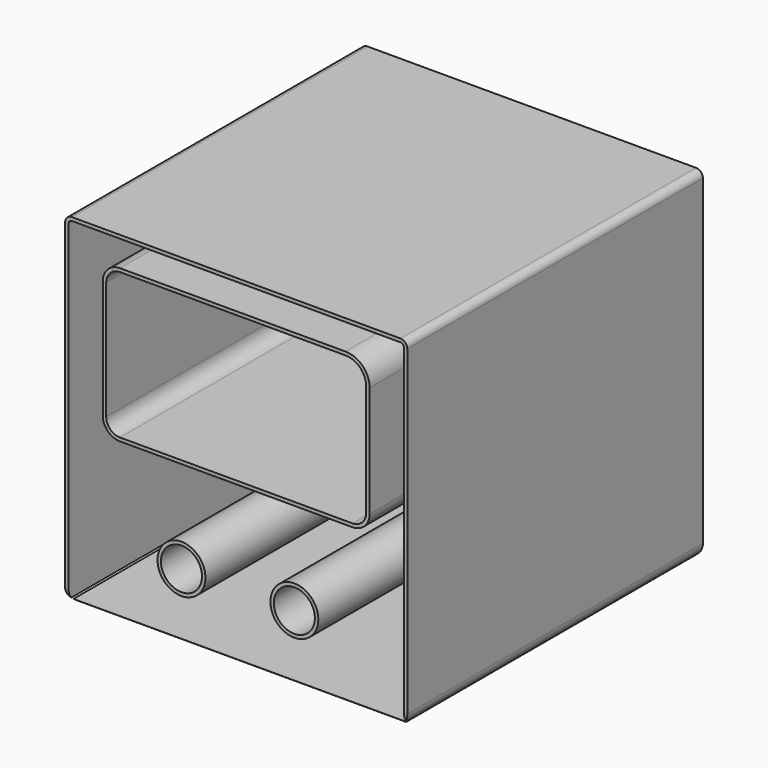
from build123d import *

# Parameters (mm, degrees)
F0_W        = 250
F0_H        = 250
F0_R        = 15
F1_DEPTH    = 20
F2_R        = 5
F3_DEPTH    = 250
F5_T        = -2.5
F6_T1_DEPTH = 45
F6_T3_DEPTH = 275
F6_T5_DEPTH = 300


# Not quite as in the source:
# - a fillet or chamfer that OpenCascade refuses, or shapes differently, is made with other operations: its cross-section is extruded or revolved along the edge and cut away or added
# - the program builds the solid bodies; features that only make, move or delete a surface that nothing else refers to are left out


with BuildPart() as f1:
    # F0 (on Front) → F1 (new body)
    with BuildSketch(Plane.XZ):
        with Locations((79.7126553953, -72.3895989358)):
            Rectangle(F0_W, F0_H)
        with Locations((39.7126553953, -147.645547986)):
            Circle(F0_R, mode=Mode.SUBTRACT)
        with Locations((122.2126553953, -147.645547986)):
            Circle(F0_R, mode=Mode.SUBTRACT)
        with BuildLine():
            Line((-15.2873446047, -67.7264088296), (-15.2873446047, 18.6264493965))
            ThreePointArc((-15.2873446047, 18.6264493965), (-12.3539628579, 25.7082593932), (-5.2721528612, 28.64164114))
            Line((-5.2721528612, 28.64164114), (159.5934226625, 28.64164114))
            ThreePointArc((159.5934226625, 28.64164114), (170.2843346542, 24.2133203989), (174.7126553953, 13.5224084073))
            Line((174.7126553953, 13.5224084073), (174.7126553953, -67.7264088296))
            ThreePointArc((174.7126553953, -67.7264088296), (171.7792736485, -74.8082188263), (164.6974636518, -77.7416005731))
            Line((164.6974636518, -77.7416005731), (-5.2721528612, -77.7416005731))
            ThreePointArc((-5.2721528612, -77.7416005731), (-12.3539628579, -74.8082188263), (-15.2873446047, -67.7264088296))
        make_face(mode=Mode.SUBTRACT)
    extrude(amount=F1_DEPTH)

    # F2
    f2_edges = [f1.edges().sort_by_distance(p)[0] for p in [
        (204.712655, -10, 52.610401),
        (-45.287345, -10, 52.610401),
    ]]
    fillet(f2_edges, radius=F2_R)

    # F3 (add): a face of the model
    f3_faces = [f1.faces().sort_by_distance(p)[0] for p in [
        (79.7304888538, -20, -93.2584337022),
    ]]
    extrude(f3_faces, amount=F3_DEPTH)

    # F5
    f5_openings = [f1.faces().sort_by_distance(p)[0] for p in [
        (79.730489, -270, -93.258434),
    ]]
    offset(amount=F5_T, openings=f5_openings, kind=Kind.INTERSECTION)

    # F6: fillet of radius 10 on 5 edges, made by hand

    # F6_s2 → F6_t1 (cut)
    with BuildSketch(Plane.XZ.offset(-25)):
        with BuildLine():
            ThreePointArc((204.7126553953, -187.3895989358), (201.7837232071, -194.4606667477), (194.7126553953, -197.3895989358))
            Line((194.7126553953, -197.3895989358), (204.7126553953, -197.3895989358))
            Line((204.7126553953, -197.3895989358), (204.7126553953, -187.3895989358))
        make_face()
        with BuildLine():
            ThreePointArc((-35.2873446047, -197.3895989358), (-42.3584124166, -194.4606667477), (-45.2873446047, -187.3895989358))
            Line((-45.2873446047, -187.3895989358), (-45.2873446047, -197.3895989358))
            Line((-45.2873446047, -197.3895989358), (-35.2873446047, -197.3895989358))
        make_face()
    extrude(amount=F6_T1_DEPTH, mode=Mode.SUBTRACT)

    # F6_s4 → F6_t3 (cut)
    with BuildSketch(Plane.XZ.offset(20)):
        with BuildLine():
            ThreePointArc((204.7126553953, -187.3895989358), (201.7837232071, -194.4606667477), (194.7126553953, -197.3895989358))
            Line((194.7126553953, -197.3895989358), (204.7126553953, -197.3895989358))
            Line((204.7126553953, -197.3895989358), (204.7126553953, -187.3895989358))
        make_face()
        with BuildLine():
            ThreePointArc((-35.2873446047, -197.3895989358), (-42.3584124166, -194.4606667477), (-45.2873446047, -187.3895989358))
            Line((-45.2873446047, -187.3895989358), (-45.2873446047, -197.3895989358))
            Line((-45.2873446047, -197.3895989358), (-35.2873446047, -197.3895989358))
        make_face()
    extrude(amount=F6_T3_DEPTH, mode=Mode.SUBTRACT)

    # F6_s6 → F6_t5 (cut)
    with BuildSketch(Plane.YZ.offset(-70.2873446047)):
        with BuildLine():
            ThreePointArc((-260, -197.3895989358), (-267.0710678119, -194.4606667477), (-270, -187.3895989358))
            Line((-270, -187.3895989358), (-270, -197.3895989358))
            Line((-270, -197.3895989358), (-260, -197.3895989358))
        make_face()
    extrude(amount=F6_T5_DEPTH, mode=Mode.SUBTRACT)


solid = f1.part
